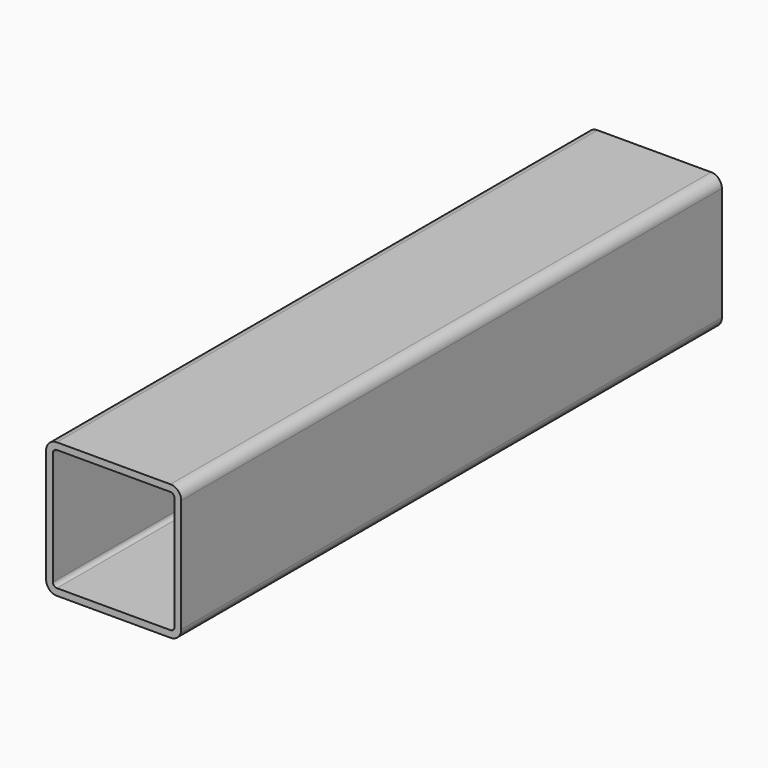
from build123d import *

# Parameters (mm, degrees)
F1_DEPTH = 250


# Not quite as in the source:
# - a feature names something its author has since deleted; it is built from what else it names


with BuildPart() as f1:
    # F0 (on Front) → F1 (new body)
    with BuildSketch(Plane.XZ):
        with BuildLine():
            Line((21, 25), (-21, 25))
            ThreePointArc((-21, 25), (-23.8284271247, 23.8284271247), (-25, 21))
            Line((-25, 21), (-25, -21))
            ThreePointArc((-25, -21), (-23.8284271247, -23.8284271247), (-21, -25))
            Line((-21, -25), (21, -25))
            ThreePointArc((21, -25), (23.8284271247, -23.8284271247), (25, -21))
            Line((25, -21), (25, 21))
            ThreePointArc((25, 21), (23.8284271247, 23.8284271247), (21, 25))
        make_face()
        with BuildLine():
            ThreePointArc((-22.5, 21), (-22.0606601718, 22.0606601718), (-21, 22.5))
            Line((-21, 22.5), (21, 22.5))
            ThreePointArc((21, 22.5), (22.0606601718, 22.0606601718), (22.5, 21))
            Line((22.5, 21), (22.5, -21))
            ThreePointArc((22.5, -21), (22.0606601718, -22.0606601718), (21, -22.5))
            Line((21, -22.5), (-21, -22.5))
            ThreePointArc((-21, -22.5), (-22.0606601718, -22.0606601718), (-22.5, -21))
            Line((-22.5, -21), (-22.5, 21))
        make_face(mode=Mode.SUBTRACT)
    extrude(amount=F1_DEPTH)


solid = f1.part
